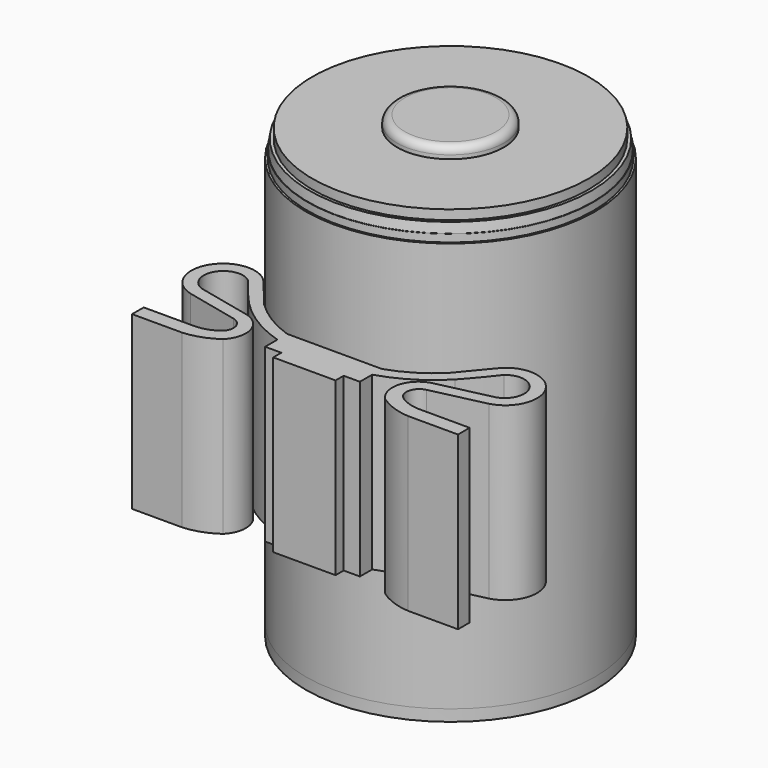
from build123d import *

# Parameters (mm, degrees)
F2_DEPTH       = 45
F4_R           = 38
F5_DEPTH       = 55.25
F7_DEPTH       = 45
F8_R           = 37.5
F9_DEPTH       = 2
F10_R          = 37.4
F11_DEPTH      = 2.5
F11_TAPER      = 8
F11_DEPTH_BACK = 25
F12_R          = 36.25
F13_DEPTH      = 2.5
F14_R          = 14
F5_FACE1_R     = 38
F15_DEPTH      = 3
F16_R          = 2


with BuildPart() as f2:
    # F1 (on Top) → F2 (new body)
    with BuildSketch(Plane.XY):
        with BuildLine():
            Line((-42.7623353899, 4.772992339), (-42.7623353899, 0.9551661788))
            Line((-42.7623353899, 0.9551661788), (-29.6120457351, 0.9551661788))
            ThreePointArc((-29.6120457351, 0.9551661788), (-25.2633665331, 1.8643256085), (-21.3180668652, 3.9069200866))
            ThreePointArc((-21.3180668652, 3.9069200866), (-19.4726981458, 10.6806652344), (-24.5569021704, 15.5221400588))
            Line((-24.5569021704, 15.5221400588), (-38.5941788554, 18.7059398741))
            ThreePointArc((-38.5941788554, 18.7059398741), (-41.3879536384, 26.1139438263), (-33.5937328637, 27.5045633316))
            ThreePointArc((-33.5937328637, 27.5045633316), (-30.4010264003, 23.5282383436), (-27.0505733788, 19.6838919073))
            ThreePointArc((-27.0505733788, 19.6838919073), (-14.6826563319, 11.4803283735), (0, 9.3162050471))
            ThreePointArc((0, 9.3162050471), (14.6826563319, 11.4803283735), (27.0505733788, 19.6838919073))
            ThreePointArc((27.0505733788, 19.6838919073), (30.4010264003, 23.5282383436), (33.5937328637, 27.5045633316))
            ThreePointArc((33.5937328637, 27.5045633316), (41.3879536384, 26.1139438263), (38.5941788554, 18.7059398741))
            Line((38.5941788554, 18.7059398741), (24.5569021704, 15.5221400588))
            ThreePointArc((24.5569021704, 15.5221400588), (19.4726981458, 10.6806652344), (21.3180668652, 3.9069200866))
            ThreePointArc((21.3180668652, 3.9069200866), (25.2633665331, 1.8643256085), (29.6120457351, 0.9551661788))
            Line((29.6120457351, 0.9551661788), (42.7623353899, 0.9551661788))
            Line((42.7623353899, 0.9551661788), (42.7623353899, 4.772992339))
            Line((42.7623353899, 4.772992339), (29.6120457351, 4.772992339))
            ThreePointArc((29.6120457351, 4.772992339), (26.3691321778, 5.3282354057), (23.4956573695, 6.9307102822))
            ThreePointArc((23.4956573695, 6.9307102822), (22.8570637764, 10.1739231369), (25.3019461508, 12.3985088452))
            Line((25.3019461508, 12.3985088452), (39.1790941358, 15.57139121))
            ThreePointArc((39.1790941358, 15.57139121), (44.369461521, 27.5896469324), (31.4749777317, 29.8503264785))
            ThreePointArc((31.4749777317, 29.8503264785), (27.8210747764, 25.4860510297), (24.2009833455, 21.0936889052))
            ThreePointArc((24.2009833455, 21.0936889052), (13.0370554513, 14.1423064512), (0, 12.4130900949))
            ThreePointArc((0, 12.4130900949), (-13.0370554513, 14.1423064512), (-24.2009833455, 21.0936889052))
            ThreePointArc((-24.2009833455, 21.0936889052), (-27.8210747764, 25.4860510297), (-31.4749777317, 29.8503264785))
            ThreePointArc((-31.4749777317, 29.8503264785), (-44.369461521, 27.5896469324), (-39.1790941358, 15.57139121))
            Line((-39.1790941358, 15.57139121), (-25.3019461508, 12.3985088452))
            ThreePointArc((-25.3019461508, 12.3985088452), (-22.8570637764, 10.1739231369), (-23.4956573695, 6.9307102822))
            ThreePointArc((-23.4956573695, 6.9307102822), (-26.3691321778, 5.3282354057), (-29.6120457351, 4.772992339))
            Line((-29.6120457351, 4.772992339), (-42.7623353899, 4.772992339))
        make_face()
    extrude(amount=F2_DEPTH)

    # F6 (on face) → F7 (join)
    with BuildSketch(Plane.XY.offset(45)):
        Polygon((12.4345744927, 6.6851694137), (12.4345744927, 13.9331343145), (-12.4345744927, 13.9478761571), (-12.4345744927, 6.6851694137), (-8.1776473671, 6.6851694137), (-8.1776473671, 4.027030806), (8.1776473671, 4.027030806), (8.1776473671, 6.6851694137), align=None)
    extrude(amount=-F7_DEPTH)


with BuildPart() as f5:
    # F4 (on offset) → F5 (new body, symmetric)
    with BuildSketch(Plane.XY.offset(19)):
        with Locations((0, 51.9405119121)):
            Circle(F4_R)
    extrude(amount=F5_DEPTH, both=True)


with BuildPart() as f9:
    # F8 (on face) → F9 (new body)
    with BuildSketch(Plane.XY.offset(74.25)):
        with Locations((0, 51.9405119121)):
            Circle(F8_R)
    extrude(amount=F9_DEPTH)

    # F10 (on face) → F11 (join, two sides)
    with BuildSketch(Plane.XY.offset(76.25)) as f11_sk:
        with Locations((0, 51.9405119121)):
            Circle(F10_R)
    extrude(amount=F11_DEPTH, taper=F11_TAPER)
    extrude(f11_sk.sketch, amount=-F11_DEPTH_BACK)

    # F12 (on face) → F13 (join)
    with BuildSketch(Plane.XY.offset(78.75)):
        with Locations((0, 51.9405119121)):
            Circle(F12_R)
    extrude(amount=F13_DEPTH)

    # F14 (on face) + F5_face1 (on face) → F15 (join)
    with BuildSketch(Plane.XY.offset(81.25)):
        with Locations((0, 51.9405119121)):
            Circle(F14_R)
    with BuildSketch(Plane(origin=(0, 51.9405119121, -36.25), x_dir=(1, 0, 0), z_dir=(0, 0, -1))):
        Circle(F5_FACE1_R)
    extrude(amount=F15_DEPTH, dir=(0, 0, 1))

    # F16
    f16_edges = [f9.edges().sort_by_distance(p)[0] for p in [
        (-14, 51.940512, 84.25),
    ]]
    fillet(f16_edges, radius=F16_R)


solid = Compound([f2.part, f5.part, f9.part])
